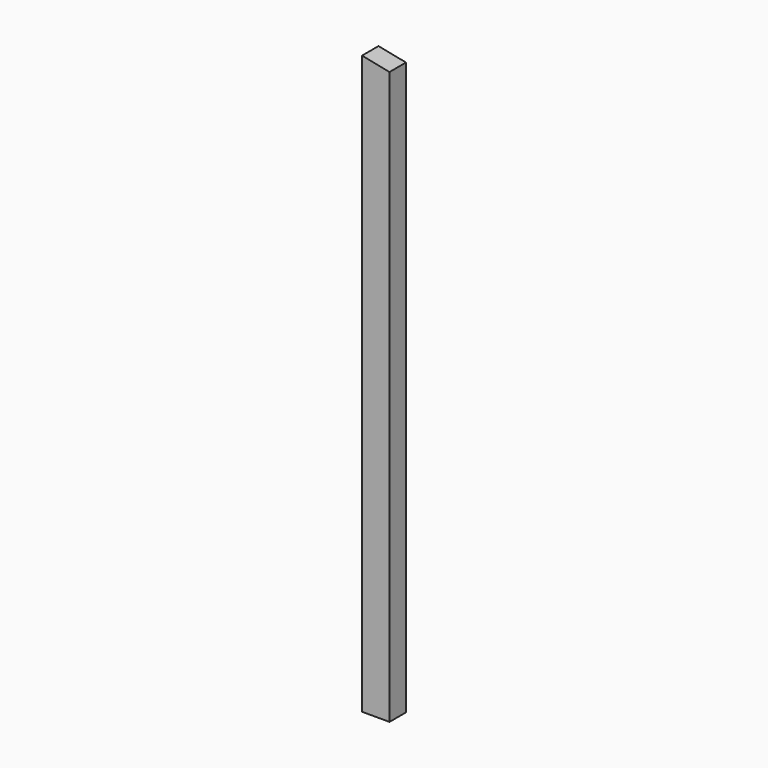
from build123d import *

# Parameters (mm, degrees)
F0_W     = 100
F0_H     = 75
F1_DEPTH = 2100
F2_SIZE2 = 19.981962
F2_SIZE  = 99.99999


# Not quite as in the source:
# - a fillet or chamfer is up to 0.001 mm smaller than in the source, because OpenCascade refuses the exact size


with BuildPart() as f1:
    # F0 (on Top) → F1 (new body)
    with BuildSketch(Plane.XY):
        with Locations((-50, -37.5)):
            Rectangle(F0_W, F0_H)
    extrude(amount=F1_DEPTH)

    # F2 (size 100 and 19.9819717699 in the source; OpenCascade refuses exactly that, so slightly less here)
    f2_edges = [f1.edges().sort_by_distance(p)[0] for p in [
        (0, -37.5, 2100),
    ]]
    f2_side = f1.faces().sort_by_distance((-50, -37.5, 2100))[0]
    chamfer(f2_edges, length=F2_SIZE, length2=F2_SIZE2, reference=f2_side)


solid = f1.part
